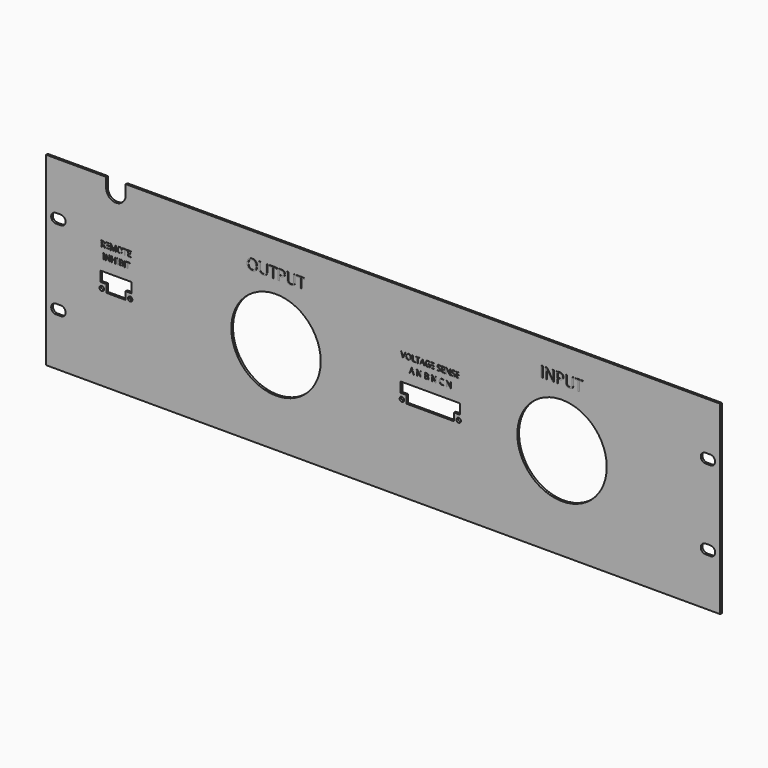
from build123d import *

# Parameters (mm, degrees)
F1_DEPTH        = 1.5
F2_DEPTH        = 1.5
F3_W            = 3.5
F3_H            = 6.8
F4_W            = 3.5
F4_H            = 6.8
F5_W            = 3.5
F5_H            = 6.8
F6_W            = 3.5
F6_H            = 6.8
F7_DEPTH        = 3
F8_R            = 32
F8_R_2          = 1.6
F8_R_3          = 1.6002
F9_DEPTH        = 3
F10_TEXT_SIZE   = 10.5833333333
F10_TEXT_SIZE_2 = 5.5639574372
F10_TEXT_SIZE_3 = 5.5738888889
F11_DEPTH       = 0.254


# Not quite as in the source:
# - Text() gives the source's letters only with a copy of the font that has no kerning and outlines rounded to 1/6400 em; it was checked with that copy


with BuildPart() as f1:
    # F0 (on Front) → F1 (new body)
    with BuildSketch(Plane.XZ):
        with BuildLine():
            Line((-198.3, 66.3), (-241.3, 66.3))
            Line((-241.3, 66.3), (-241.3, -66.3))
            Line((-241.3, -66.3), (241.3, -66.3))
            Line((241.3, -66.3), (241.3, 66.3))
            Line((241.3, 66.3), (-184.3, 66.3))
            Line((-184.3, 66.3), (-184.3, 59.3))
            ThreePointArc((-184.3, 59.3), (-191.3, 52.3), (-198.3, 59.3))
            Line((-198.3, 59.3), (-198.3, 66.3))
        make_face()
        with BuildLine():
            Line((-184.3, 66.3), (-198.3, 66.3))
            Line((-198.3, 66.3), (-198.3, 59.3))
            ThreePointArc((-198.3, 59.3), (-191.3, 52.3), (-184.3, 59.3))
            Line((-184.3, 59.3), (-184.3, 66.3))
        make_face()
    extrude(amount=-F1_DEPTH)

    # F0 (on Front) → F2 (cut)
    with BuildSketch(Plane.XZ):
        with BuildLine():
            Line((-184.3, 66.3), (-198.3, 66.3))
            Line((-198.3, 66.3), (-198.3, 59.3))
            ThreePointArc((-198.3, 59.3), (-191.3, 52.3), (-184.3, 59.3))
            Line((-184.3, 59.3), (-184.3, 66.3))
        make_face()
    extrude(amount=-F2_DEPTH, mode=Mode.SUBTRACT)

    # F3 (on face) + F4 (on face) + F5 (on face) + F6 (on face) → F7 (cut)
    with BuildSketch(Plane.XZ):
        with Locations((-232.5, 28.6)):
            Rectangle(F3_W, F3_H)
        with BuildLine():
            Line((-230.75, 32), (-230.75, 25.2))
            ThreePointArc((-230.75, 25.2), (-227.35, 28.6), (-230.75, 32))
        make_face()
        with BuildLine():
            ThreePointArc((-234.25, 32), (-237.65, 28.6), (-234.25, 25.2))
            Line((-234.25, 25.2), (-234.25, 32))
        make_face()
    with BuildSketch(Plane.XZ):
        with Locations((-232.5, -28.6)):
            Rectangle(F4_W, F4_H)
        with BuildLine():
            Line((-230.75, -25.2), (-230.75, -32))
            ThreePointArc((-230.75, -32), (-227.35, -28.6), (-230.75, -25.2))
        make_face()
        with BuildLine():
            ThreePointArc((-234.25, -25.2), (-237.65, -28.6), (-234.25, -32))
            Line((-234.25, -32), (-234.25, -25.2))
        make_face()
    with BuildSketch(Plane.XZ):
        with Locations((232.5, 28.6)):
            Rectangle(F5_W, F5_H)
        with BuildLine():
            ThreePointArc((234.25, 25.2), (237.65, 28.6), (234.25, 32))
            Line((234.25, 32), (234.25, 25.2))
        make_face()
        with BuildLine():
            Line((230.75, 25.2), (230.75, 32))
            ThreePointArc((230.75, 32), (227.35, 28.6), (230.75, 25.2))
        make_face()
    with BuildSketch(Plane.XZ):
        with Locations((232.5, -28.6)):
            Rectangle(F6_W, F6_H)
        with BuildLine():
            Line((234.25, -25.2), (234.25, -32))
            ThreePointArc((234.25, -32), (237.65, -28.6), (234.25, -25.2))
        make_face()
        with BuildLine():
            ThreePointArc((230.75, -25.2), (227.35, -28.6), (230.75, -32))
            Line((230.75, -32), (230.75, -25.2))
        make_face()
    extrude(amount=-F7_DEPTH, mode=Mode.SUBTRACT)

    # F8 (on face) → F9 (cut)
    with BuildSketch(Plane.XZ):
        with Locations((-76.7, 0)):
            Circle(F8_R)
        with Locations((128.05, 0)):
            Circle(F8_R)
        Polygon((54.83, -1.2), (54.83, 6), (12.58, 6), (12.58, -1.2), (16.705, -1.2), (16.705, -6.7), (50.705, -6.7), (50.705, -1.2), align=None)
        with Locations((54.04, -5)):
            Circle(F8_R_2)
        with Locations((13.4, -5)):
            Circle(F8_R_2)
        Polygon((-180.3, -1.2), (-180.3, 6), (-202.3, 6), (-202.3, -1.2), (-198.15, -1.2), (-198.15, -6.7), (-184.45, -6.7), (-184.45, -1.2), align=None)
        with Locations((-181.14, -5)):
            Circle(F8_R_3)
        with Locations((-201.46, -5)):
            Circle(F8_R_3)
    extrude(amount=-F9_DEPTH, mode=Mode.SUBTRACT)

    # F10 (on face) → F11 (join)
    with BuildSketch(Plane.XZ):
        with Locations((-97.8600520833, 41.3)):
            Text('OUTPUT', F10_TEXT_SIZE, font='Open Sans', text_align=(TextAlign.LEFT, TextAlign.BOTTOM))
        with Locations((112.3263085938, 41.3)):
            Text('INPUT', F10_TEXT_SIZE, font='Open Sans', text_align=(TextAlign.LEFT, TextAlign.BOTTOM))
        with Locations((12.58, 21.3)):
            Text('VOLTAGE SENSE', F10_TEXT_SIZE_2, font='Open Sans', text_align=(TextAlign.LEFT, TextAlign.BOTTOM))
        with Locations((18.5407640625, 13.2736)):
            Text('A N B N C N', F10_TEXT_SIZE_3, font='Open Sans', text_align=(TextAlign.LEFT, TextAlign.BOTTOM))
        with Locations((-202.3641694444, 21.3)):
            Text('REMOTE', F10_TEXT_SIZE_3, font='Open Sans', text_align=(TextAlign.LEFT, TextAlign.BOTTOM))
        with Locations((-200.9158292535, 13.7195111111)):
            Text('INHIBIT', F10_TEXT_SIZE_3, font='Open Sans', text_align=(TextAlign.LEFT, TextAlign.BOTTOM))
    extrude(amount=F11_DEPTH)


solid = f1.part
